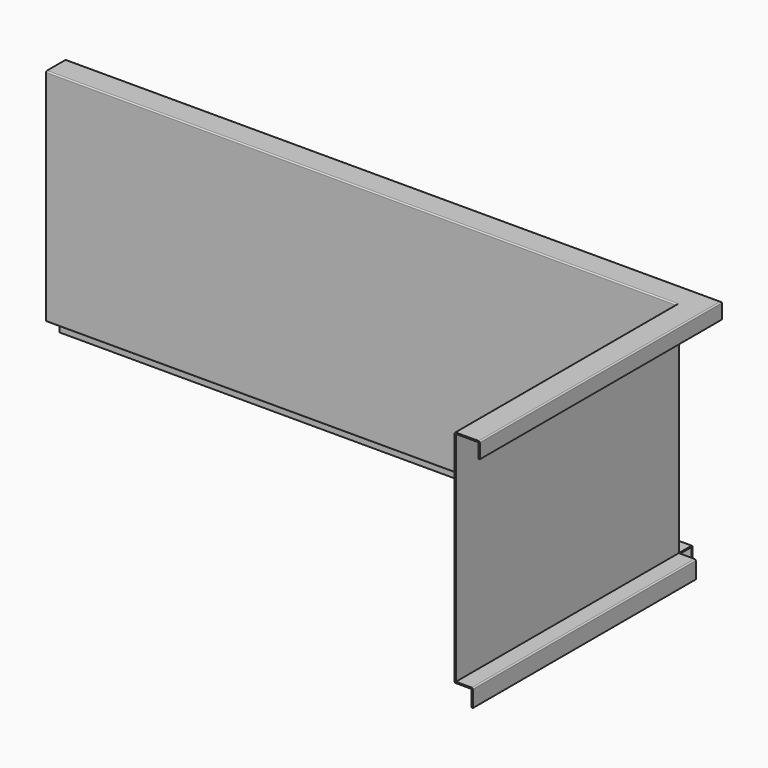
from build123d import *

# Parameters (mm, degrees)
F3_W         = 27
F3_H         = 27
F4_DEPTH     = 30
F5_T1_DEPTH  = 1002
F5_T3_DEPTH  = 1038
F5_T5_DEPTH  = 442
F5_T7_DEPTH  = 478
F5_T13_DEPTH = 447
F5_T17_DEPTH = 1007
F5_T20_DEPTH = 1012
F5_T22_DEPTH = 1050
F5_T24_DEPTH = 1005
F5_T26_DEPTH = 445
F5_T28_DEPTH = 490
F5_T30_DEPTH = 452
F5_T36_DEPTH = 1010
F5_T40_DEPTH = 450
F5_T47_DEPTH = 1010
F5_T51_DEPTH = 450


# Not quite as in the source:
# - a fillet or chamfer that OpenCascade refuses, or shapes differently, is made with other operations: its cross-section is extruded or revolved along the edge and cut away or added


with BuildPart() as f2:
    # F2: sweep along a path in F1
    with BuildLine(Plane.XY) as f2_path:
        Line((0, 0), (0, 440))
        Line((0, 440), (-1000, 440))
    # F0 (on Front) → F2 (sweep)
    with BuildSketch(Plane.XZ):
        Polygon((38, -2), (38, -25), (40, -25), (40, 0), (0, 0), (0, -350), (27, -350), (27, -376), (29, -376), (29, -348), (2, -348), (2, -2), align=None)
    sweep(path=f2_path.line, transition=Transition.RIGHT)

    # F3 (on face) → F4 (cut)
    with BuildSketch(Plane.XY.offset(-348)):
        with Locations((15.5, 455.5)):
            Rectangle(F3_W, F3_H)
    extrude(amount=-F4_DEPTH, mode=Mode.SUBTRACT)

    # F5: fillet of radius 2 on 15 edges, made by hand

    # F5_s2 → F5_t1 (join)
    with BuildSketch(Plane.YZ.offset(-1000)):
        with BuildLine():
            ThreePointArc((442, -346), (442.5857864376, -347.4142135624), (444, -348))
            Line((444, -348), (442, -348))
            Line((442, -348), (442, -346))
        make_face()
        with BuildLine():
            ThreePointArc((465, -350), (466.4142135624, -350.5857864376), (467, -352))
            Line((467, -352), (467, -350))
            Line((467, -350), (465, -350))
        make_face()
        with BuildLine():
            ThreePointArc((444, -2), (442.5857864376, -2.5857864376), (442, -4))
            Line((442, -4), (442, -2))
            Line((442, -2), (444, -2))
        make_face()
    extrude(amount=F5_T1_DEPTH)

    # F5_s4 → F5_t3 (join)
    with BuildSketch(Plane.YZ.offset(-1000)):
        with BuildLine():
            ThreePointArc((476, -2), (477.4142135624, -2.5857864376), (478, -4))
            Line((478, -4), (478, -2))
            Line((478, -2), (476, -2))
        make_face()
    extrude(amount=F5_T3_DEPTH)

    # F5_s6 → F5_t5 (join)
    with BuildSketch(Plane.XZ.offset(-442)):
        with BuildLine():
            ThreePointArc((25, -350), (26.4142135624, -350.5857864376), (27, -352))
            Line((27, -352), (27, -350))
            Line((27, -350), (25, -350))
        make_face()
        with BuildLine():
            ThreePointArc((4, -2), (2.5857864376, -2.5857864376), (2, -4))
            Line((2, -4), (2, -2))
            Line((2, -2), (4, -2))
        make_face()
    extrude(amount=F5_T5_DEPTH)

    # F5_s8 → F5_t7 (join)
    with BuildSketch(Plane.XZ.offset(-478)):
        with BuildLine():
            ThreePointArc((38, -4), (37.4142135624, -2.5857864376), (36, -2))
            Line((36, -2), (38, -2))
            Line((38, -2), (38, -4))
        make_face()
    extrude(amount=F5_T7_DEPTH)


with BuildPart() as f5_tool11:
    # F5_s12 → F5_t13 (new body)
    with BuildSketch(Plane.XZ):
        with BuildLine():
            ThreePointArc((4, -2), (2.5857864376, -2.5857864376), (2, -4))
            Line((2, -4), (2, -2))
            Line((2, -2), (4, -2))
        make_face()
    extrude(amount=-F5_T13_DEPTH)

    split(bisect_by=Plane.XZ.offset(-442), keep=Keep.BOTTOM)


with BuildPart() as f5_tool15:
    # F5_s16 → F5_t17 (new body)
    with BuildSketch(Plane.YZ.offset(7)):
        with BuildLine():
            ThreePointArc((444, -2), (442.5857864376, -2.5857864376), (442, -4))
            Line((442, -4), (442, -2))
            Line((442, -2), (444, -2))
        make_face()
    extrude(amount=-F5_T17_DEPTH)

    split(bisect_by=Plane.YZ.offset(2), keep=Keep.TOP)


with BuildPart() as f5_tool11_1:
    add(f5_tool11.part)

    # F5_t19: intersect F5_tool15
    add(f5_tool15.part, mode=Mode.INTERSECT)


with BuildPart() as f2_1:
    add(f2.part)

    # F5_t9: union F5_tool11
    add(f5_tool11_1.part)

    # F5_s21 → F5_t20 (cut)
    with BuildSketch(Plane.YZ.offset(-1005)):
        with BuildLine():
            ThreePointArc((467, -348), (468.4142135624, -348.5857864376), (469, -350))
            Line((469, -350), (469, -348))
            Line((469, -348), (467, -348))
        make_face()
    extrude(amount=F5_T20_DEPTH, mode=Mode.SUBTRACT)

    # F5_s23 → F5_t22 (cut)
    with BuildSketch(Plane.YZ.offset(-1005)):
        with BuildLine():
            ThreePointArc((480, -2), (479.4142135624, -0.5857864376), (478, 0))
            Line((478, 0), (480, 0))
            Line((480, 0), (480, -2))
        make_face()
    extrude(amount=F5_T22_DEPTH, mode=Mode.SUBTRACT)

    # F5_s25 → F5_t24 (cut)
    with BuildSketch(Plane.YZ.offset(-1005)):
        with BuildLine():
            ThreePointArc((440, -2), (440.5857864376, -0.5857864376), (442, 0))
            Line((442, 0), (440, 0))
            Line((440, 0), (440, -2))
        make_face()
        with BuildLine():
            ThreePointArc((440, -348), (440.5857864376, -349.4142135624), (442, -350))
            Line((442, -350), (440, -350))
            Line((440, -350), (440, -348))
        make_face()
    extrude(amount=F5_T24_DEPTH, mode=Mode.SUBTRACT)

    # F5_s27 → F5_t26 (cut)
    with BuildSketch(Plane.XZ.offset(-440)):
        with BuildLine():
            ThreePointArc((0, -2), (0.5857864376, -0.5857864376), (2, 0))
            Line((2, 0), (0, 0))
            Line((0, 0), (0, -2))
        make_face()
        with BuildLine():
            ThreePointArc((2, -350), (0.5857864376, -349.4142135624), (0, -348))
            Line((0, -348), (0, -350))
            Line((0, -350), (2, -350))
        make_face()
    extrude(amount=F5_T26_DEPTH, mode=Mode.SUBTRACT)

    # F5_s29 → F5_t28 (cut)
    with BuildSketch(Plane.XZ.offset(-485)):
        with BuildLine():
            ThreePointArc((38, 0), (39.4142135624, -0.5857864376), (40, -2))
            Line((40, -2), (40, 0))
            Line((40, 0), (38, 0))
        make_face()
    extrude(amount=F5_T28_DEPTH, mode=Mode.SUBTRACT)

    # F5_s31 → F5_t30 (cut)
    with BuildSketch(Plane.XZ.offset(-447)):
        with BuildLine():
            ThreePointArc((27, -348), (28.4142135624, -348.5857864376), (29, -350))
            Line((29, -350), (29, -348))
            Line((29, -348), (27, -348))
        make_face()
    extrude(amount=F5_T30_DEPTH, mode=Mode.SUBTRACT)


with BuildPart() as f5_tool34:
    # F5_s35 → F5_t36 (new body)
    with BuildSketch(Plane.YZ.offset(5)):
        with BuildLine():
            ThreePointArc((440, -2), (440.5857864376, -0.5857864376), (442, 0))
            Line((442, 0), (440, 0))
            Line((440, 0), (440, -2))
        make_face()
    extrude(amount=-F5_T36_DEPTH)

    split(bisect_by=Plane.YZ, keep=Keep.TOP)


with BuildPart() as f5_tool38:
    # F5_s39 → F5_t40 (new body)
    with BuildSketch(Plane.XZ.offset(5)):
        with BuildLine():
            ThreePointArc((0, -2), (0.5857864376, -0.5857864376), (2, 0))
            Line((2, 0), (0, 0))
            Line((0, 0), (0, -2))
        make_face()
    extrude(amount=-F5_T40_DEPTH)

    split(bisect_by=Plane.XZ.offset(-440), keep=Keep.BOTTOM)


with BuildPart() as f5_tool34_1:
    add(f5_tool34.part)

    # F5_t42: intersect F5_tool38
    add(f5_tool38.part, mode=Mode.INTERSECT)


with BuildPart() as f2_2:
    add(f2_1.part)

    # F5_t32: cut F5_tool34
    add(f5_tool34_1.part, mode=Mode.SUBTRACT)


with BuildPart() as f5_tool45:
    # F5_s46 → F5_t47 (new body)
    with BuildSketch(Plane.YZ.offset(5)):
        with BuildLine():
            ThreePointArc((440, -348), (440.5857864376, -349.4142135624), (442, -350))
            Line((442, -350), (440, -350))
            Line((440, -350), (440, -348))
        make_face()
    extrude(amount=-F5_T47_DEPTH)

    split(bisect_by=Plane.YZ, keep=Keep.TOP)


with BuildPart() as f5_tool49:
    # F5_s50 → F5_t51 (new body)
    with BuildSketch(Plane.XZ.offset(5)):
        with BuildLine():
            ThreePointArc((2, -350), (0.5857864376, -349.4142135624), (0, -348))
            Line((0, -348), (0, -350))
            Line((0, -350), (2, -350))
        make_face()
    extrude(amount=-F5_T51_DEPTH)

    split(bisect_by=Plane.XZ.offset(-440), keep=Keep.BOTTOM)


with BuildPart() as f5_tool45_1:
    add(f5_tool45.part)

    # F5_t53: intersect F5_tool49
    add(f5_tool49.part, mode=Mode.INTERSECT)


with BuildPart() as f2_3:
    add(f2_2.part)

    # F5_t43: cut F5_tool45
    add(f5_tool45_1.part, mode=Mode.SUBTRACT)


solid = f2_3.part
